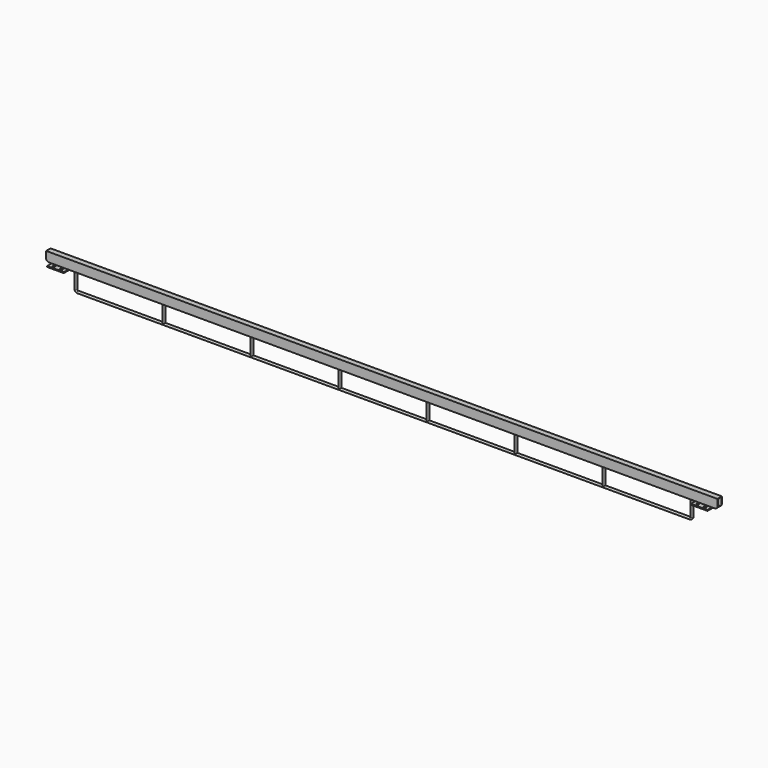
from build123d import *

# Parameters (mm, degrees)
F0_W          = 3575
F0_H          = 50
F1_DEPTH      = 15
F1_DEPTH_BACK = 15
F3_DEPTH      = 5
F5_DEPTH      = 5
F6_R          = 6
F7_DEPTH      = 5
F8_R          = 6
F9_DEPTH      = 5
F10_R         = 6
F21_DEPTH     = 5
F22_W         = 30
F22_H         = 50
F23_DEPTH     = 30
F24_R         = 15
F25_W         = 26
F25_H         = 13
F25_H_2       = 33
F26_DEPTH     = 100
F27_W         = 30
F27_H         = 50
F28_DEPTH     = 30
F29_W         = 26
F29_H         = 46
F30_DEPTH     = 100
F31_T1_DEPTH  = 105


# Not quite as in the source:
# - a fillet or chamfer that OpenCascade refuses, or shapes differently, is made with other operations: its cross-section is extruded or revolved along the edge and cut away or added


with BuildPart() as f1:
    # F0 (on Front) → F1 (new body, two sides)
    with BuildSketch(Plane.XZ) as f1_sk:
        Rectangle(F0_W, F0_H)
    extrude(amount=F1_DEPTH)
    extrude(f1_sk.sketch, amount=-F1_DEPTH_BACK)

    # F2 (on face) → F3 (join)
    with BuildSketch(Plane(origin=(0, 0, -25), x_dir=(1, 0, 0), z_dir=(0, 0, -1))):
        Polygon((-1787.5, 45), (-1787.5, 15), (-1787.5, -15), (-1697.5, -15), (-1697.5, 45), align=None)
    extrude(amount=F3_DEPTH)

    # F4 (on face) → F5 (join)
    with BuildSketch(Plane(origin=(0, 0, -25), x_dir=(1, 0, 0), z_dir=(0, 0, -1))):
        Polygon((1787.5, -15), (1787.5, 15), (1787.5, 45), (1697.5, 45), (1697.5, -15), align=None)
    extrude(amount=F5_DEPTH)

    # F6 (on face) → F7 (cut, through all)
    with BuildSketch(Plane(origin=(0, 0, -30), x_dir=(1, 0, 0), z_dir=(0, 0, -1))):
        with Locations((-935, 30)):
            Circle(F6_R)
        with Locations((-975, 30)):
            Circle(F6_R)
    extrude(amount=-F7_DEPTH, mode=Mode.SUBTRACT)

    # F8 (on face) → F9 (cut, through all)
    with BuildSketch(Plane(origin=(0, 0, -30), x_dir=(1, 0, 0), z_dir=(0, 0, -1))):
        with Locations((1762.5, 30)):
            Circle(F8_R)
        with Locations((1722.5, 30)):
            Circle(F8_R)
    extrude(amount=-F9_DEPTH, mode=Mode.SUBTRACT)

    # F12: sweep along a path in F11
    with BuildLine(Plane.XZ) as f12_path:
        Line((-1667.5, -25), (-1667.5, -115))
        ThreePointArc((-1667.5, -115), (-1664.5710678119, -122.0710678119), (-1657.5, -125))
        Line((-1657.5, -125), (1657.5, -125))
        ThreePointArc((1657.5, -125), (1664.5710678119, -122.0710678119), (1667.5, -115))
        Line((1667.5, -115), (1667.5, -25))
    # F10 (on face) → F12 (sweep)
    with BuildSketch(Plane(origin=(0, 0, -25), x_dir=(1, 0, 0), z_dir=(0, 0, -1))):
        with Locations((-1667.5, 0)):
            Circle(F10_R)
    sweep(path=f12_path.line)

    # F13: sweep along a path in F11
    with BuildLine(Plane.XZ) as f13_path:
        Line((-1191.0714285714, -25), (-1191.0714285714, -125))
    # F10 (on face) → F13 (sweep)
    with BuildSketch(Plane(origin=(0, 0, -25), x_dir=(1, 0, 0), z_dir=(0, 0, -1))):
        with BuildLine():
            Line((-1191.0714285714, 0), (-1197.0714285714, 0))
            ThreePointArc((-1197.0714285714, 0), (-1191.0714285714, -6), (-1185.0714285714, 0))
            Line((-1185.0714285714, 0), (-1191.0714285714, 0))
        make_face()
        with BuildLine():
            ThreePointArc((-1185.0714285714, 0), (-1191.0714285714, 6), (-1197.0714285714, 0))
            Line((-1197.0714285714, 0), (-1191.0714285714, 0))
            Line((-1191.0714285714, 0), (-1185.0714285714, 0))
        make_face()
    sweep(path=f13_path.line)

    # F14: sweep along a path in F11
    with BuildLine(Plane.XZ) as f14_path:
        Line((-714.6428571429, -25), (-714.6428571429, -125))
    # F10 (on face) → F14 (sweep)
    with BuildSketch(Plane(origin=(0, 0, -25), x_dir=(1, 0, 0), z_dir=(0, 0, -1))):
        with BuildLine():
            ThreePointArc((-708.6428571429, 0), (-714.6428571429, 6), (-720.6428571429, 0))
            Line((-720.6428571429, 0), (-714.6428571429, 0))
            Line((-714.6428571429, 0), (-708.6428571429, 0))
        make_face()
        with BuildLine():
            Line((-714.6428571429, 0), (-720.6428571429, 0))
            ThreePointArc((-720.6428571429, 0), (-714.6428571429, -6), (-708.6428571429, 0))
            Line((-708.6428571429, 0), (-714.6428571429, 0))
        make_face()
    sweep(path=f14_path.line)

    # F15: sweep along a path in F11
    with BuildLine(Plane.XZ) as f15_path:
        Line((-238.2142857143, -25), (-238.2142857143, -125))
    # F10 (on face) → F15 (sweep)
    with BuildSketch(Plane(origin=(0, 0, -25), x_dir=(1, 0, 0), z_dir=(0, 0, -1))):
        with BuildLine():
            ThreePointArc((-232.2142857143, 0), (-238.2142857143, 6), (-244.2142857143, 0))
            Line((-244.2142857143, 0), (-238.2142857143, 0))
            Line((-238.2142857143, 0), (-232.2142857143, 0))
        make_face()
        with BuildLine():
            Line((-238.2142857143, 0), (-244.2142857143, 0))
            ThreePointArc((-244.2142857143, 0), (-238.2142857143, -6), (-232.2142857143, 0))
            Line((-232.2142857143, 0), (-238.2142857143, 0))
        make_face()
    sweep(path=f15_path.line)

    # F16: sweep along a path in F11
    with BuildLine(Plane.XZ) as f16_path:
        Line((-1667.5, -25), (-1667.5, -115))
        ThreePointArc((-1667.5, -115), (-1664.5710678119, -122.0710678119), (-1657.5, -125))
        Line((-1657.5, -125), (1657.5, -125))
        ThreePointArc((1657.5, -125), (1664.5710678119, -122.0710678119), (1667.5, -115))
    # F10 (on face) → F16 (sweep)
    with BuildSketch(Plane(origin=(0, 0, -25), x_dir=(1, 0, 0), z_dir=(0, 0, -1))):
        with Locations((-1667.5, 0)):
            Circle(F10_R)
    sweep(path=f16_path.line)

    # F17: sweep along a path in F11
    with BuildLine(Plane.XZ) as f17_path:
        Line((238.2142857143, -25), (238.2142857143, -125))
    # F10 (on face) → F17 (sweep)
    with BuildSketch(Plane(origin=(0, 0, -25), x_dir=(1, 0, 0), z_dir=(0, 0, -1))):
        with BuildLine():
            ThreePointArc((244.2142857143, 0), (238.2142857143, 6), (232.2142857143, 0))
            Line((232.2142857143, 0), (238.2142857143, 0))
            Line((238.2142857143, 0), (244.2142857143, 0))
        make_face()
        with BuildLine():
            Line((238.2142857143, 0), (232.2142857143, 0))
            ThreePointArc((232.2142857143, 0), (238.2142857143, -6), (244.2142857143, 0))
            Line((244.2142857143, 0), (238.2142857143, 0))
        make_face()
    sweep(path=f17_path.line)

    # F18: sweep along a path in F11
    with BuildLine(Plane.XZ) as f18_path:
        Line((714.6428571429, -25), (714.6428571429, -125))
    # F10 (on face) → F18 (sweep)
    with BuildSketch(Plane(origin=(0, 0, -25), x_dir=(1, 0, 0), z_dir=(0, 0, -1))):
        with BuildLine():
            ThreePointArc((720.6428571429, 0), (714.6428571429, 6), (708.6428571429, 0))
            Line((708.6428571429, 0), (714.6428571429, 0))
            Line((714.6428571429, 0), (720.6428571429, 0))
        make_face()
        with BuildLine():
            Line((714.6428571429, 0), (708.6428571429, 0))
            ThreePointArc((708.6428571429, 0), (714.6428571429, -6), (720.6428571429, 0))
            Line((720.6428571429, 0), (714.6428571429, 0))
        make_face()
    sweep(path=f18_path.line)

    # F19: sweep along a path in F11
    with BuildLine(Plane.XZ) as f19_path:
        Line((1191.0714285714, -25), (1191.0714285714, -125))
    # F10 (on face) → F19 (sweep)
    with BuildSketch(Plane(origin=(0, 0, -25), x_dir=(1, 0, 0), z_dir=(0, 0, -1))):
        with BuildLine():
            Line((1191.0714285714, 0), (1185.0714285714, 0))
            ThreePointArc((1185.0714285714, 0), (1191.0714285714, -6), (1197.0714285714, 0))
            Line((1197.0714285714, 0), (1191.0714285714, 0))
        make_face()
        with BuildLine():
            ThreePointArc((1197.0714285714, 0), (1191.0714285714, 6), (1185.0714285714, 0))
            Line((1185.0714285714, 0), (1191.0714285714, 0))
            Line((1191.0714285714, 0), (1197.0714285714, 0))
        make_face()
    sweep(path=f19_path.line)

    # F20 (on face) → F21 (cut, through all)
    with BuildSketch(Plane(origin=(0, 0, -30), x_dir=(1, 0, 0), z_dir=(0, 0, -1))):
        with BuildLine():
            ThreePointArc((-1762.5, 36), (-1766.7426406871, 34.2426406871), (-1768.5, 30))
            Line((-1768.5, 30), (-1762.5, 30))
            Line((-1762.5, 30), (-1762.5, 36))
        make_face()
        with BuildLine():
            ThreePointArc((-1716.5, 30), (-1722.5, 36), (-1728.5, 30))
            ThreePointArc((-1728.5, 30), (-1722.5, 24), (-1716.5, 30))
        make_face()
        with BuildLine():
            Line((-1762.5, 30), (-1768.5, 30))
            ThreePointArc((-1768.5, 30), (-1762.5, 24), (-1756.5, 30))
            Line((-1756.5, 30), (-1762.5, 30))
        make_face()
        with BuildLine():
            Line((-1762.5, 36), (-1762.5, 30))
            Line((-1762.5, 30), (-1756.5, 30))
            ThreePointArc((-1756.5, 30), (-1758.2573593129, 34.2426406871), (-1762.5, 36))
        make_face()
    extrude(amount=-F21_DEPTH, mode=Mode.SUBTRACT)

    # F22 (on face) → F23 (join)
    with BuildSketch(Plane.YZ.offset(1787.5)):
        Rectangle(F22_W, F22_H)
    extrude(amount=F23_DEPTH)

    # F24
    f24_edges = [f1.edges().sort_by_distance(p)[0] for p in [
        (1817.5, 0, -25),
    ]]
    fillet(f24_edges, radius=F24_R)

    # F25 (on face) → F26 (cut)
    with BuildSketch(Plane.YZ.offset(1817.5)):
        with Locations((0, -16.5)):
            Rectangle(F25_W, F25_H)
        with Locations((0, 6.5)):
            Rectangle(F25_W, F25_H_2)
    extrude(amount=-F26_DEPTH, mode=Mode.SUBTRACT)

    # F27 (on face) → F28 (join)
    with BuildSketch(Plane(origin=(-1787.5, 0, 0), x_dir=(0, -1, 0), z_dir=(-1, 0, 0))):
        Rectangle(F27_W, F27_H)
    extrude(amount=F28_DEPTH)

    # F29 (on face) → F30 (cut)
    with BuildSketch(Plane(origin=(-1817.5, 0, 0), x_dir=(0, -1, 0), z_dir=(-1, 0, 0))):
        Rectangle(F29_W, F29_H)
    extrude(amount=-F30_DEPTH, mode=Mode.SUBTRACT)

    # F31: fillet of radius 15 on 1 edges, made by hand

    # F31_s2 → F31_t1 (cut)
    with BuildSketch(Plane.XZ.offset(-52.5)):
        with BuildLine():
            ThreePointArc((-1817.5, -10), (-1813.1066017178, -20.6066017178), (-1802.5, -25))
            Line((-1802.5, -25), (-1817.5, -25))
            Line((-1817.5, -25), (-1817.5, -10))
        make_face()
    extrude(amount=F31_T1_DEPTH, mode=Mode.SUBTRACT)


solid = f1.part
